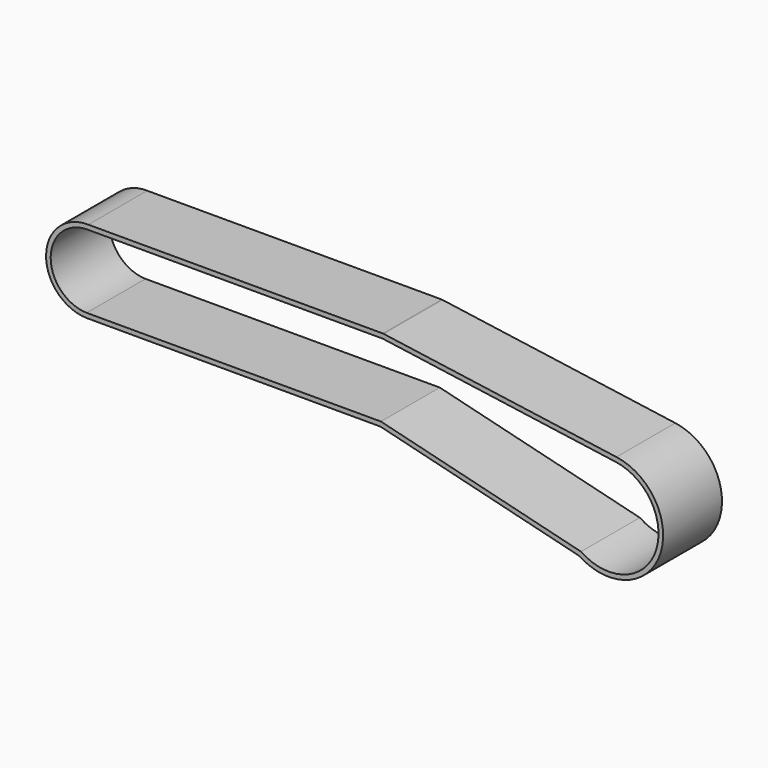
from build123d import *

# Parameters (mm, degrees)
F1_DEPTH = 20


# Not quite as in the source:
# - ends of sketch curves that miss each other by under 0.0002 mm in the source are joined


with BuildPart() as f1:
    # F0 (on Front) → F1 (new body)
    with BuildSketch(Plane.XZ):
        with BuildLine():
            Line((97.2907843779, 1.1145511836), (34.0001858397, 10.009464731))
            Line((34.0001858397, 10.009464731), (33.8270701172, 10.0337945591))
            Line((33.8270701172, 10.0337945591), (33.7396616023, 10.0337945591))
            Line((33.7396616023, 10.0337945591), (-46.2468009406, 10.0337945591))
            ThreePointArc((-46.2468009406, 10.0337945591), (-57.7296417452, -0.9784425912), (-46.7174045949, -12.4612833958))
            Line((-46.7174045949, -12.4612833958), (33.1437814598, -12.4612833958))
            Line((33.1437814598, -12.4612833958), (87.1445596341, -25.8231245195))
            ThreePointArc((87.1445596341, -25.8231245195), (109.0413090103, -18.6910027208), (97.2907843779, 1.1145511836))
        make_face()
        with BuildLine():
            ThreePointArc((-46.7038671765, -11.2112851433), (-56.4796434927, -0.9919800096), (-46.260338359, 8.7837963066))
            Line((-46.260338359, 8.7837963066), (33.7396616023, 8.7837945591))
            Line((33.7396616023, 8.7837945591), (97.1168180017, -0.1232839023))
            ThreePointArc((97.1168180017, -0.1232839023), (107.8343480434, -18.3479856965), (87.6567253878, -24.6621562401))
            Line((87.6567253878, -24.6621562401), (33.2961328623, -11.2112833958))
            Line((33.2961328623, -11.2112833958), (-46.7038671765, -11.2112851433))
        make_face(mode=Mode.SUBTRACT)
    extrude(amount=F1_DEPTH)


solid = f1.part
